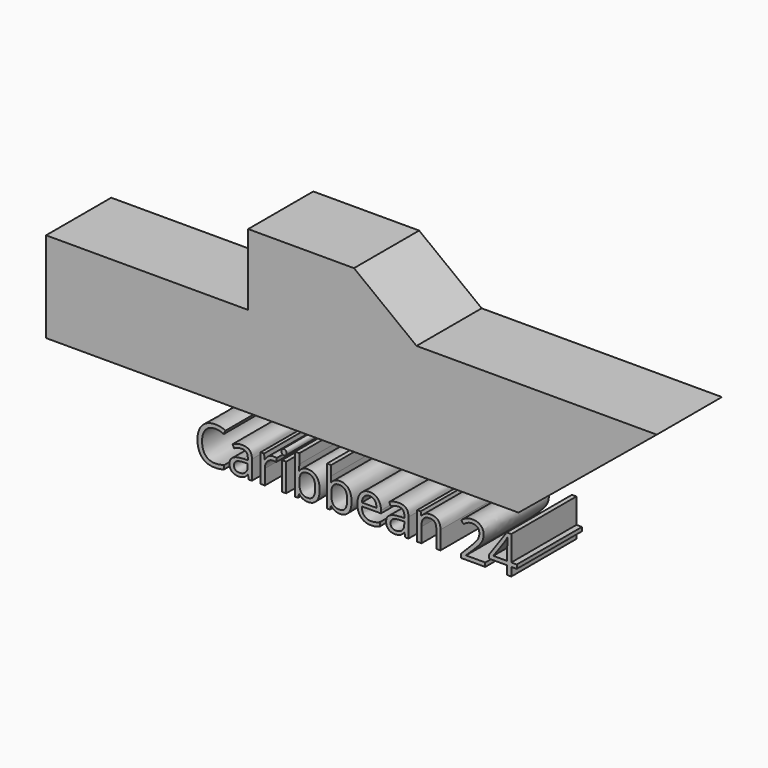
from build123d import *

# Parameters (mm, degrees)
F0_TEXT_SIZE = 25.6040030056
F1_DEPTH     = 40


# Not quite as in the source:
# - Text() gives the source's letters only with a copy of the font that has no kerning and outlines rounded to 1/6400 em; it was checked with that copy


with BuildPart() as f1:
    # F0 (on Front) → F1 (new body)
    with BuildSketch(Plane.XZ):
        Polygon((0, -120.8771020174), (0, -165.3345823288), (232.0903539658, -165.3345823288), (300, -109.5325648785), (181.9853037596, -109.5325648785), (151.260510087, -85.8981087804), (99.2647111416, -85.8981087804), (99.2647111416, -120.8771020174), align=None)
        with Locations((72.7941207588, -194.1439062357)):
            Text('Caribbean 24', F0_TEXT_SIZE, font='Open Sans', text_align=(TextAlign.LEFT, TextAlign.BOTTOM))
    extrude(amount=F1_DEPTH)


solid = f1.part
